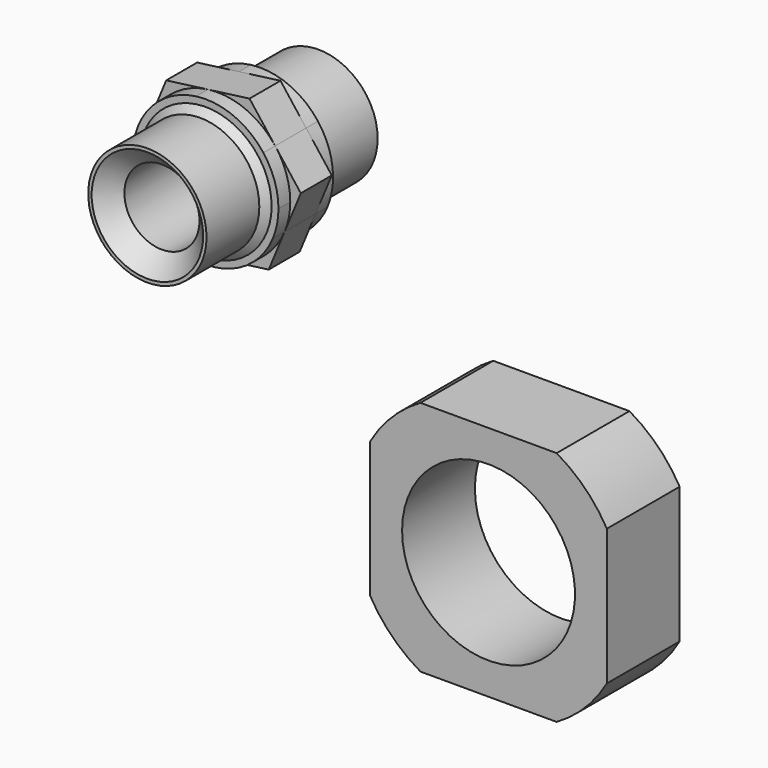
from build123d import *

# Parameters (mm, degrees)
F0_R     = 15
F1_DEPTH = 20
F2_D     = 38
F2_DEPTH = 20
F2_TIP   = 11.416352
F3_R     = 13
F3_R_2   = 8.25
F4_DEPTH = 23.5
F5_DEPTH = 7.5
F6_DEPTH = 4.25
F7_SIZE  = 4
F8_SIZE  = 4
F9_SIZE  = 1.5


with BuildPart() as f1:
    # F0 (on Front) → F1 (new body)
    with BuildSketch(Plane.XZ):
        with BuildLine():
            ThreePointArc((26, 14.96663), (21.213203, 21.213203), (14.96663, 26))
            Line((14.96663, 26), (-14.96663, 26))
            ThreePointArc((-14.96663, 26), (-21.213203, 21.213203), (-26, 14.96663))
            Line((-26, 14.96663), (-26, -14.96663))
            ThreePointArc((-26, -14.96663), (-21.213203, -21.213203), (-14.96663, -26))
            Line((-14.96663, -26), (14.96663, -26))
            ThreePointArc((14.96663, -26), (21.213203, -21.213203), (26, -14.96663))
            Line((26, -14.96663), (26, 14.96663))
        make_face()
        Circle(F0_R, mode=Mode.SUBTRACT)
        Circle(F0_R)
    extrude(amount=F1_DEPTH)

    # F2
    with Locations(Plane(origin=(0, 0, 0), x_dir=(1, 0, 0), z_dir=(0, 1, 0))):
        with Locations((0, 0)):
            Hole(F2_D / 2, depth=F2_DEPTH)
            with Locations((0, 0, -(F2_DEPTH + F2_TIP / 2))):  # 118° drill point
                Cone(0, F2_D / 2, F2_TIP, mode=Mode.SUBTRACT)


with BuildPart() as f4:
    # F3 (on Front) → F4 (new body, symmetric)
    with BuildSketch(Plane.XZ):
        with Locations((-72.170123, 45.066312)):
            Circle(F3_R)
        with Locations((-72.170123, 45.066312)):
            Circle(F3_R_2, mode=Mode.SUBTRACT)
    extrude(amount=F4_DEPTH, both=True)

    # F3 (on Front) → F5 (join, symmetric)
    with BuildSketch(Plane.XZ):
        with BuildLine():
            ThreePointArc((-70.065855, 29.205289), (-62.417262, 32.382397), (-57.38194, 38.958151))
            ThreePointArc((-57.38194, 38.958151), (-56.476001, 41.952707), (-56.170123, 45.066312))
            ThreePointArc((-56.170123, 45.066312), (-57.021813, 50.216912), (-59.486209, 54.819173))
            ThreePointArc((-59.486209, 54.819173), (-66.061962, 59.854495), (-74.274392, 60.927335))
            ThreePointArc((-74.274392, 60.927335), (-81.922985, 57.750227), (-86.958307, 51.174474))
            ThreePointArc((-86.958307, 51.174474), (-88.031147, 42.962043), (-84.854038, 35.31345))
            ThreePointArc((-84.854038, 35.31345), (-78.278285, 30.278129), (-70.065855, 29.205289))
        make_face()
        with Locations((-72.170123, 45.066312)):
            Circle(F3_R, mode=Mode.SUBTRACT)
    extrude(amount=F5_DEPTH, both=True)

    # F3 (on Front) → F6 (join, symmetric)
    with BuildSketch(Plane.XZ):
        with BuildLine():
            Line((-60.908489, 30.420189), (-57.38194, 38.958151))
            ThreePointArc((-57.38194, 38.958151), (-62.417262, 32.382397), (-70.065855, 29.205289))
            Line((-70.065855, 29.205289), (-60.908489, 30.420189))
        make_face()
        with BuildLine():
            Line((-79.223221, 27.990389), (-70.065855, 29.205289))
            ThreePointArc((-70.065855, 29.205289), (-78.278285, 30.278129), (-84.854038, 35.31345))
            Line((-84.854038, 35.31345), (-79.223221, 27.990389))
        make_face()
        with BuildLine():
            Line((-90.484855, 42.636512), (-84.854038, 35.31345))
            ThreePointArc((-84.854038, 35.31345), (-88.031147, 42.962043), (-86.958307, 51.174474))
            Line((-86.958307, 51.174474), (-90.484855, 42.636512))
        make_face()
        with BuildLine():
            ThreePointArc((-86.958307, 51.174474), (-81.922985, 57.750227), (-74.274392, 60.927335))
            Line((-74.274392, 60.927335), (-83.431758, 59.712435))
            Line((-83.431758, 59.712435), (-86.958307, 51.174474))
        make_face()
        with BuildLine():
            ThreePointArc((-74.274392, 60.927335), (-66.061962, 59.854495), (-59.486209, 54.819173))
            Line((-59.486209, 54.819173), (-65.117026, 62.142235))
            Line((-65.117026, 62.142235), (-74.274392, 60.927335))
        make_face()
        with BuildLine():
            Line((-57.38194, 38.958151), (-53.855392, 47.496112))
            Line((-53.855392, 47.496112), (-59.486209, 54.819173))
            ThreePointArc((-59.486209, 54.819173), (-57.021813, 50.216912), (-56.170123, 45.066312))
            ThreePointArc((-56.170123, 45.066312), (-56.476001, 41.952707), (-57.38194, 38.958151))
        make_face()
    extrude(amount=F6_DEPTH, both=True)

    # F7
    f7_edges = [f4.edges().sort_by_distance(p)[0] for p in [
        (-80.420123, -23.5, 45.066312),
    ]]
    chamfer(f7_edges, length=F7_SIZE)

    # F8
    f8_edges = [f4.edges().sort_by_distance(p)[0] for p in [
        (-80.420123, 23.5, 45.066312),
    ]]
    chamfer(f8_edges, length=F8_SIZE)

    # F9
    f9_edges = [f4.edges().sort_by_distance(p)[0] for p in [
        (-85.170123, 7.5, 45.066312),
        (-85.170123, -7.5, 45.066312),
    ]]
    chamfer(f9_edges, length=F9_SIZE)


solid = Compound([f1.part, f4.part])
